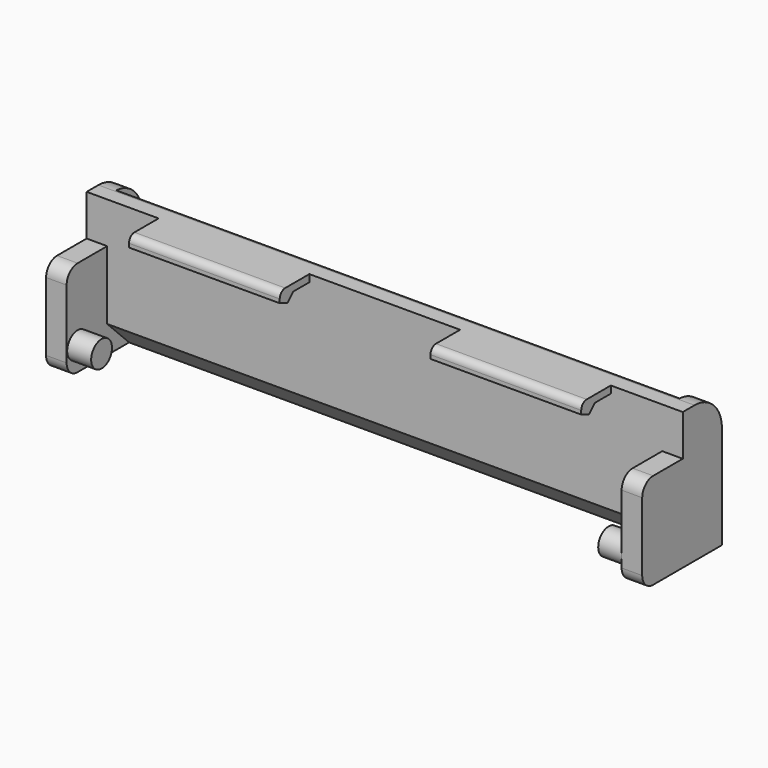
from build123d import *

# Parameters (mm, degrees)
F1_DEPTH  = 3
F3_DEPTH  = 17
F5_DEPTH  = 17.6
F6_W      = 3
F6_H      = 14
F7_DEPTH  = 7.4
F8_R      = 2
F6_W_2    = 22
F6_H_2    = 2.1
F9_DEPTH  = 5.4
F10_R     = 1
F12_SIZE  = 4
F14_DEPTH = 3.5
F18_DEPTH = 66
F20_DEPTH = 4.7397795647
F21_F1_R  = 4.9999


# Not quite as in the source:
# - a fillet or chamfer is up to 0.001 mm smaller than in the source, because OpenCascade refuses the exact size


with BuildPart() as f1:
    # F0 (on Top) → F1 (new body)
    with BuildSketch(Plane.XY):
        with BuildLine():
            Line((43.5, -20), (43.5, 0))
            ThreePointArc((43.5, 0), (20.8194176131, -3.2823932686), (0, -12.8602204353))
            Line((0, -12.8602204353), (0, -20))
            Line((0, -20), (43.5, -20))
        make_face()
        with BuildLine():
            ThreePointArc((87, -12.8602204353), (66.1805823869, -3.2823932686), (43.5, 0))
            Line((43.5, 0), (43.5, -20))
            Line((43.5, -20), (87, -20))
            Line((87, -20), (87, -12.8602204353))
        make_face()
    extrude(amount=F1_DEPTH)

    # F2 (on face) → F3 (join)
    with BuildSketch(Plane.XY.offset(3)):
        with BuildLine():
            ThreePointArc((87, -12.8602204353), (43.5, 0), (0, -12.8602204353))
            Line((0, -12.8602204353), (0, -20))
            Line((0, -20), (87, -20))
            Line((87, -20), (87, -12.8602204353))
        make_face()
        with BuildLine():
            Line((84.6, -17.6), (2.4, -17.6))
            Line((2.4, -17.6), (2.4, -14.1778912523))
            ThreePointArc((2.4, -14.1778912523), (43.5, -2.4), (84.6, -14.1778912523))
            Line((84.6, -14.1778912523), (84.6, -17.6))
        make_face(mode=Mode.SUBTRACT)
    extrude(amount=F3_DEPTH)

    # F4 (on Front) → F5 (cut, through all)
    with BuildSketch(Plane.XZ):
        with BuildLine():
            ThreePointArc((130.5, 90), (-18.0182899632, 151.5182899632), (43.5, 3))
            ThreePointArc((43.5, 3), (105.0182899632, 28.4817100368), (130.5, 90))
        make_face()
    extrude(amount=F5_DEPTH, mode=Mode.SUBTRACT)

    # F6 (on face) → F7 (join)
    with BuildSketch(Plane.XZ.offset(20)):
        with Locations((1.5, 7)):
            Rectangle(F6_W, F6_H)
        with Locations((85.5, 7)):
            Rectangle(F6_W, F6_H)
    extrude(amount=F7_DEPTH)

    # F8
    f8_edges = [f1.edges().sort_by_distance(p)[0] for p in [
        (1.5, -27.4, 0),
        (1.5, -27.4, 14),
        (85.5, -27.4, 14),
        (85.5, -27.4, 0),
    ]]
    fillet(f8_edges, radius=F8_R)

    # F6 (on face) → F9 (join)
    with BuildSketch(Plane.XZ.offset(20)):
        with Locations((21.5, 18.95)):
            Rectangle(F6_W_2, F6_H_2)
        with Locations((65.5, 18.95)):
            Rectangle(F6_W_2, F6_H_2)
    extrude(amount=F9_DEPTH)

    # F10
    f10_edges = [f1.edges().sort_by_distance(p)[0] for p in [
        (21.5, -25.4, 20),
        (65.5, -25.4, 20),
    ]]
    fillet(f10_edges, radius=F10_R)

    # F12
    f12_edges = [f1.edges().sort_by_distance(p)[0] for p in [
        (43.5, -20, 0),
    ]]
    chamfer(f12_edges, length=F12_SIZE)

    # F13 (on face) → F14 (join)
    with BuildSketch(Plane.YZ.offset(3)):
        with BuildLine():
            Line((-25.4, 2), (-26.566190379, 2))
            ThreePointArc((-26.566190379, 2), (-26.0164414003, 1.7027799244), (-25.4, 1.6))
            Line((-25.4, 1.6), (-25.4, 2))
        make_face()
        with BuildLine():
            ThreePointArc((-23.5, 3.5), (-26.2349366084, 5.2067163971), (-26.566190379, 2))
            Line((-26.566190379, 2), (-25.4, 2))
            Line((-25.4, 2), (-25.4, 1.6))
            ThreePointArc((-25.4, 1.6), (-24.0564971157, 2.1564971157), (-23.5, 3.5))
        make_face()
    extrude(amount=F14_DEPTH)

    # F17: F1 across plane


with BuildPart() as f1_1:
    add(f1.part)
    add(f1.part.mirror(Plane.YZ.offset(43.5)))

    # F11 (on face) → F18 (cut, through all)
    with BuildSketch(Plane(origin=(10.5, 0, 0), x_dir=(0, -1, 0), z_dir=(-1, 0, 0))):
        Polygon((22.95, 18.95), (20, 18.95), (20, 17.9), (24, 17.9), align=None)
        Polygon((25.4, 17.9), (25.4, 18.45), (24, 17.9), align=None)
    extrude(amount=-F18_DEPTH, mode=Mode.SUBTRACT)

    # F19 (on face) → F20 (join, through all)
    with BuildSketch(Plane(origin=(0, -17.6, 0), x_dir=(-1, 0, 0), z_dir=(0, 1, 0))):
        with BuildLine():
            Line((-84.6, 13.3202112679), (-84.6, 20))
            Line((-84.6, 20), (-87, 20))
            Line((-87, 20), (-87, 14.6557898708))
            ThreePointArc((-87, 14.6557898708), (-85.8052708602, 13.9785289708), (-84.6, 13.3202112679))
        make_face()
        with BuildLine():
            Line((-2.4, 20), (-2.4, 13.3202112679))
            ThreePointArc((-2.4, 13.3202112679), (-1.1947291398, 13.9785289708), (0, 14.6557898708))
            Line((0, 14.6557898708), (0, 20))
            Line((0, 20), (-2.4, 20))
        make_face()
    extrude(amount=F20_DEPTH)

    # F21: fillet of radius 5 on 2 edges, made by hand

    # F21_f1 (radius 5 in the source; OpenCascade refuses exactly that, so slightly less here)
    f21_f1_edges = [f1_1.edges().sort_by_distance(p)[0] for p in [
        (85.8, -12.8602204353, 20),
    ]]
    fillet(f21_f1_edges, radius=F21_F1_R)


solid = f1_1.part
